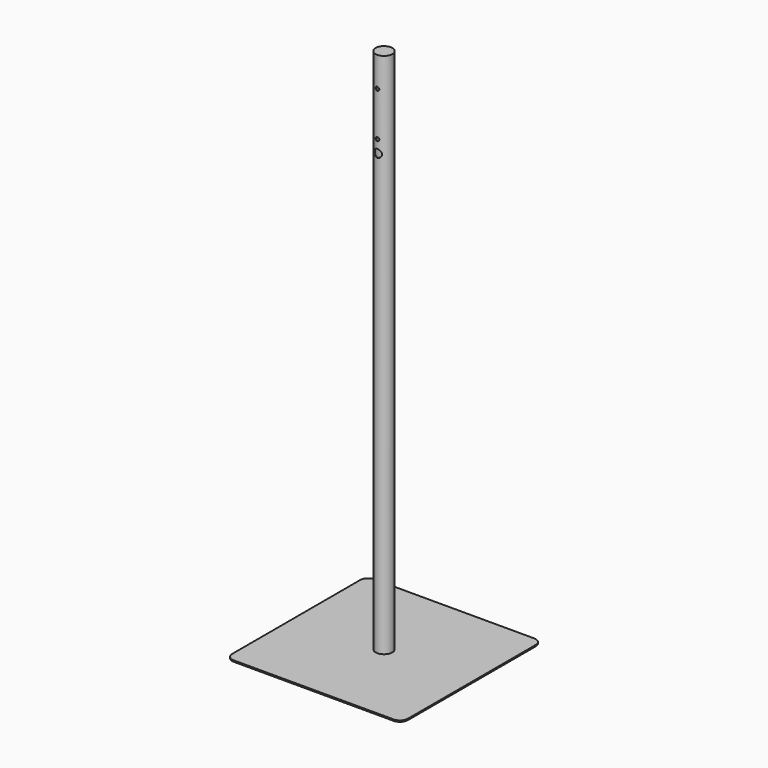
from build123d import *

# Parameters (mm, degrees)
F2_DEPTH = 19.001
F3_DEPTH = 19.0010001
F4_DEPTH = 19.0010001
F5_R     = 19
F6_DEPTH = 3
F7_R     = 19
F8_DEPTH = 3


with BuildPart() as f1:
    # F0 (on Front) → F1 (revolve)
    with BuildSketch(Plane.XZ):
        Polygon((-17.5, -43.4220433303), (-17.5, 1156.5779566697), (-19, 1156.5779566697), (-19, -41.8273694813), (-19, -43.4220433303), align=None)
    revolve(axis=Axis((0, 0, 1124.6529566697), (0, 0, -1)))

    # F0 (on Front) → F2 (cut, through all)
    with BuildSketch(Plane.XZ):
        with BuildLine():
            ThreePointArc((4.15, 987.5779566697), (2.9344931419, 990.5124498116), (0, 991.7279566697))
            ThreePointArc((0, 991.7279566697), (-4.15, 987.5779566697), (0, 983.4279566697))
            ThreePointArc((0, 983.4279566697), (2.9344931419, 984.6434635278), (4.15, 987.5779566697))
        make_face()
        with BuildLine():
            ThreePointArc((0, 967.9779566697), (-9, 958.9779566697), (0, 949.9779566697))
            ThreePointArc((0, 949.9779566697), (6.3639610307, 952.613995639), (9, 958.9779566697))
            ThreePointArc((9, 958.9779566697), (6.3639610307, 965.3419177004), (0, 967.9779566697))
        make_face()
    extrude(amount=F2_DEPTH, mode=Mode.SUBTRACT)

    # F0 (on Front) → F3 (cut, through all)
    with BuildSketch(Plane.XZ):
        with BuildLine():
            ThreePointArc((4.15, 1088.5779566697), (2.9344931419, 1091.5124498116), (0, 1092.7279566697))
            ThreePointArc((0, 1092.7279566697), (-4.15, 1088.5779566697), (0, 1084.4279566697))
            ThreePointArc((0, 1084.4279566697), (2.9344931419, 1085.6434635278), (4.15, 1088.5779566697))
        make_face()
    extrude(amount=F3_DEPTH, mode=Mode.SUBTRACT)

    # F0 (on Front) → F4 (cut, through all)
    with BuildSketch(Plane.XZ):
        with BuildLine():
            ThreePointArc((0, 967.9779566697), (-9, 958.9779566697), (0, 949.9779566697))
            ThreePointArc((0, 949.9779566697), (6.3639610307, 952.613995639), (9, 958.9779566697))
            ThreePointArc((9, 958.9779566697), (6.3639610307, 965.3419177004), (0, 967.9779566697))
        make_face()
    extrude(amount=F4_DEPTH, mode=Mode.SUBTRACT)

    # F7 (on face) → F8 (join)
    with BuildSketch(Plane.XY.offset(1156.5779566697)):
        Circle(F7_R)
    extrude(amount=-F8_DEPTH)


with BuildPart() as f6:
    # F5 (on face) → F6 (new body)
    with BuildSketch(Plane(origin=(0, 0, -43.4220433303), x_dir=(1, 0, 0), z_dir=(0, 0, -1))):
        with BuildLine():
            Line((182, 200), (-182, 200))
            ThreePointArc((-182, 200), (-194.7279220614, 194.7279220614), (-200, 182))
            Line((-200, 182), (-200, -182))
            ThreePointArc((-200, -182), (-194.7279220614, -194.7279220614), (-182, -200))
            Line((-182, -200), (182, -200))
            ThreePointArc((182, -200), (194.7279220614, -194.7279220614), (200, -182))
            Line((200, -182), (200, 182))
            ThreePointArc((200, 182), (194.7279220614, 194.7279220614), (182, 200))
        make_face()
        Circle(F5_R, mode=Mode.SUBTRACT)
    extrude(amount=F6_DEPTH)


solid = Compound([f1.part, f6.part])
